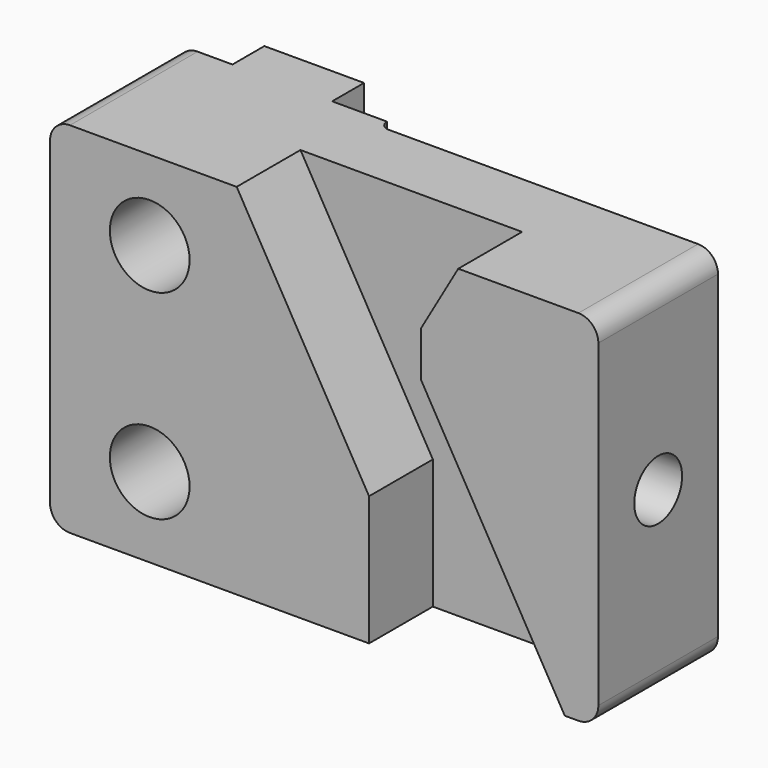
from build123d import *

# Parameters (mm, degrees)
F0_W      = 87.3125
F0_H      = 57.15
F1_DEPTH  = 31.75
F3_DEPTH  = 12.7
F4_W      = 8.73125
F4_H      = 6.35
F5_DEPTH  = 66.294
F6_R      = 1.58749
F7_R      = 3.175
F8_R      = 6.35
F9_DEPTH  = 108.204
F10_R     = 4.7625
F11_DEPTH = 12.7


# Not quite as in the source:
# - a fillet or chamfer is up to 0.001 mm smaller than in the source, because OpenCascade refuses the exact size


with BuildPart() as f1:
    # F0 (on Front) → F1 (new body)
    with BuildSketch(Plane.XZ):
        with Locations((43.65625, -28.575)):
            Rectangle(F0_W, F0_H)
    extrude(amount=F1_DEPTH)

    # F2 (on face) → F3 (cut)
    with BuildSketch(Plane.XZ.offset(31.75)):
        Polygon((50.8, -36.5125), (50.8, -57.15), (81.9624807795, -57.15), (59.048891971, -17.4625), (59.048891971, -10.31875), (65.0064250612, 0), (29.7194982962, 0), align=None)
    extrude(amount=-F3_DEPTH, mode=Mode.SUBTRACT)

    # F4 (on face) → F5 (cut)
    with BuildSketch(Plane.XY):
        Polygon((87.3125, 0), (24.60625, 0), (24.60625, -6.35), (33.3375, -6.35), (33.3375, -7.9375), (87.3125, -7.9375), align=None)
        with Locations((4.365625, -3.175)):
            Rectangle(F4_W, F4_H)
    extrude(amount=-F5_DEPTH, mode=Mode.SUBTRACT)

    # F6 (radius 1.5875 in the source; OpenCascade refuses exactly that, so slightly less here)
    f6_edges = [f1.edges().sort_by_distance(p)[0] for p in [
        (33.3375, -7.9375, -28.575),
    ]]
    fillet(f6_edges, radius=F6_R)

    # F7
    f7_edges = [f1.edges().sort_by_distance(p)[0] for p in [
        (87.3125, -19.84375, 0),
        (0, -19.05, 0),
        (87.3125, -19.84375, -57.15),
        (0, -19.05, -57.15),
    ]]
    fillet(f7_edges, radius=F7_R)

    # F8 (on face) → F9 (cut)
    with BuildSketch(Plane.XZ.offset(31.75)):
        with Locations((15.875, -12.7)):
            Circle(F8_R)
        with Locations((15.875, -44.45)):
            Circle(F8_R)
    extrude(amount=-F9_DEPTH, mode=Mode.SUBTRACT)

    # F10 (on face) → F11 (cut)
    with BuildSketch(Plane.YZ.offset(87.3125)):
        with Locations((-19.84375, -28.575)):
            Circle(F10_R)
    extrude(amount=-F11_DEPTH, mode=Mode.SUBTRACT)


solid = f1.part
